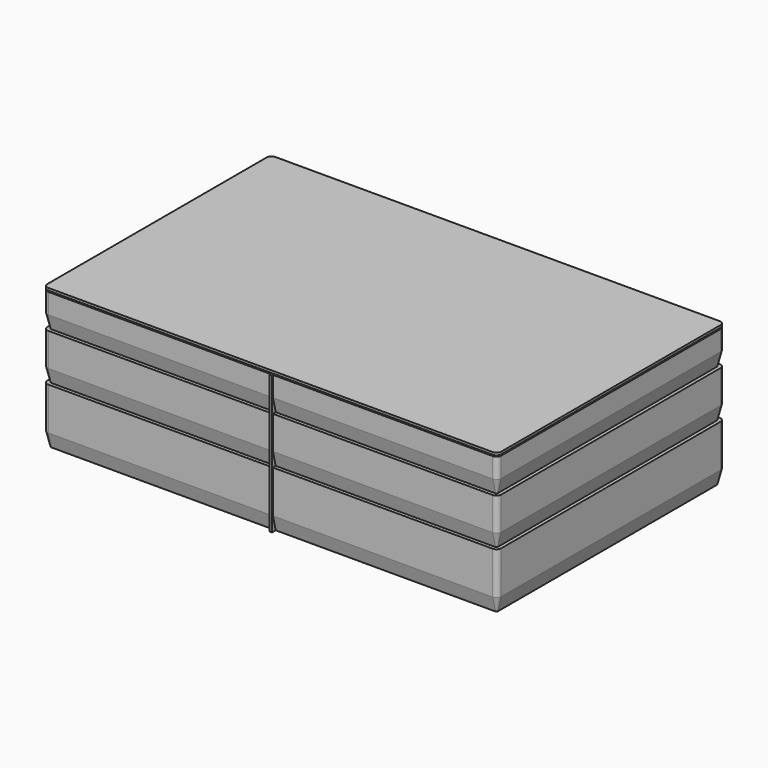
from build123d import *

# Parameters (mm, degrees)
F1_DEPTH = 6.35
F2_START = -9.525
F2_DEPTH = 92.075
F3_SIZE2 = 9.525
F3_SIZE  = 38.1
F4_START = -101.6
F4_DEPTH = 127
F5_SIZE2 = 9.525
F5_SIZE  = 38.1
F6_START = -228.6
F6_DEPTH = 152.4
F7_SIZE2 = 9.525
F7_SIZE  = 38.1
F9_START = -9.525
F8_W     = 6.35
F8_H     = 3.175
F8_H_2   = 19.05
F9_DEPTH = 371.475


# Not quite as in the source:
# - a feature names something its author has since deleted; it is built from what else it names


with BuildPart() as f1:
    # F0 (on Top) → F1 (new body)
    with BuildSketch(Plane.XY):
        with BuildLine():
            Line((39.9490956545, 736.9148339033), (-1153.8509043455, 736.9148339033))
            ThreePointArc((-1153.8509043455, 736.9148339033), (-1162.8311604666, 733.1950900244), (-1166.5509043455, 724.2148339033))
            Line((-1166.5509043455, 724.2148339033), (-1166.5509043455, 40.0023339033))
            Line((-1166.5509043455, 40.0023339033), (-1166.5509043455, 38.4148339033))
            Line((-1166.5509043455, 38.4148339033), (-1147.5009043455, 38.4148339033))
            Line((-1147.5009043455, 38.4148339033), (-1103.0509043455, 38.4148339033))
            Line((-1103.0509043455, 38.4148339033), (-1103.0509043455, -6.0351660967))
            Line((-1103.0509043455, -6.0351660967), (-1103.0509043455, -25.0851660967))
            Line((-1103.0509043455, -25.0851660967), (-1101.4634043455, -25.0851660967))
            Line((-1101.4634043455, -25.0851660967), (-560.1259043455, -25.0851660967))
            Line((-560.1259043455, -25.0851660967), (-553.7759043455, -25.0851660967))
            Line((-553.7759043455, -25.0851660967), (39.9490956545, -25.0851660967))
            ThreePointArc((39.9490956545, -25.0851660967), (48.9293517756, -21.3654222178), (52.6490956545, -12.3851660967))
            Line((52.6490956545, -12.3851660967), (52.6490956545, 724.2148339033))
            ThreePointArc((52.6490956545, 724.2148339033), (48.9293517756, 733.1950900244), (39.9490956545, 736.9148339033))
        make_face()
        with BuildLine():
            Line((-1147.5009043455, 38.4148339033), (-1166.5509043455, 38.4148339033))
            Line((-1166.5509043455, 38.4148339033), (-1166.5509043455, -12.3851660967))
            ThreePointArc((-1166.5509043455, -12.3851660967), (-1162.8311604666, -21.3654222178), (-1153.8509043455, -25.0851660967))
            Line((-1153.8509043455, -25.0851660967), (-1103.0509043455, -25.0851660967))
            Line((-1103.0509043455, -25.0851660967), (-1103.0509043455, -6.0351660967))
            Line((-1103.0509043455, -6.0351660967), (-1103.0509043455, 38.4148339033))
            Line((-1103.0509043455, 38.4148339033), (-1147.5009043455, 38.4148339033))
        make_face()
    extrude(amount=-F1_DEPTH)


with BuildPart() as f2:
    # F0 (on Top) → F2 (new body)
    with BuildSketch(Plane.XY.offset(F2_START)):
        with BuildLine():
            Line((39.9490956545, 736.9148339033), (-1153.8509043455, 736.9148339033))
            ThreePointArc((-1153.8509043455, 736.9148339033), (-1162.8311604666, 733.1950900244), (-1166.5509043455, 724.2148339033))
            Line((-1166.5509043455, 724.2148339033), (-1166.5509043455, 40.0023339033))
            Line((-1166.5509043455, 40.0023339033), (-1166.5509043455, 38.4148339033))
            Line((-1166.5509043455, 38.4148339033), (-1147.5009043455, 38.4148339033))
            Line((-1147.5009043455, 38.4148339033), (-1103.0509043455, 38.4148339033))
            Line((-1103.0509043455, 38.4148339033), (-1103.0509043455, -6.0351660967))
            Line((-1103.0509043455, -6.0351660967), (-1103.0509043455, -25.0851660967))
            Line((-1103.0509043455, -25.0851660967), (-1101.4634043455, -25.0851660967))
            Line((-1101.4634043455, -25.0851660967), (-560.1259043455, -25.0851660967))
            Line((-560.1259043455, -25.0851660967), (-553.7759043455, -25.0851660967))
            Line((-553.7759043455, -25.0851660967), (39.9490956545, -25.0851660967))
            ThreePointArc((39.9490956545, -25.0851660967), (48.9293517756, -21.3654222178), (52.6490956545, -12.3851660967))
            Line((52.6490956545, -12.3851660967), (52.6490956545, 724.2148339033))
            ThreePointArc((52.6490956545, 724.2148339033), (48.9293517756, 733.1950900244), (39.9490956545, 736.9148339033))
        make_face()
        with BuildLine():
            Line((-1147.5009043455, 38.4148339033), (-1166.5509043455, 38.4148339033))
            Line((-1166.5509043455, 38.4148339033), (-1166.5509043455, -12.3851660967))
            ThreePointArc((-1166.5509043455, -12.3851660967), (-1162.8311604666, -21.3654222178), (-1153.8509043455, -25.0851660967))
            Line((-1153.8509043455, -25.0851660967), (-1103.0509043455, -25.0851660967))
            Line((-1103.0509043455, -25.0851660967), (-1103.0509043455, -6.0351660967))
            Line((-1103.0509043455, -6.0351660967), (-1103.0509043455, 38.4148339033))
            Line((-1103.0509043455, 38.4148339033), (-1147.5009043455, 38.4148339033))
        make_face()
    extrude(amount=-F2_DEPTH)

    # F3
    f3_edges = [f2.edges().sort_by_distance(p)[0] for p in [
        (-556.950904, 736.914834, -101.6),
        (-1162.83116, 733.19509, -101.6),
        (-1166.550904, 355.914834, -101.6),
        (-1162.83116, -21.365422, -101.6),
        (-556.950904, -25.085166, -101.6),
        (48.929352, -21.365422, -101.6),
        (52.649096, 355.914834, -101.6),
        (48.929352, 733.19509, -101.6),
    ]]
    chamfer(f3_edges, length=F3_SIZE, length2=F3_SIZE2)

    # F0 (on Top) → F4 (join)
    with BuildSketch(Plane.XY.offset(F4_START)):
        with BuildLine():
            Line((39.9490956545, 736.9148339033), (-1153.8509043455, 736.9148339033))
            ThreePointArc((-1153.8509043455, 736.9148339033), (-1162.8311604666, 733.1950900244), (-1166.5509043455, 724.2148339033))
            Line((-1166.5509043455, 724.2148339033), (-1166.5509043455, 40.0023339033))
            Line((-1166.5509043455, 40.0023339033), (-1166.5509043455, 38.4148339033))
            Line((-1166.5509043455, 38.4148339033), (-1147.5009043455, 38.4148339033))
            Line((-1147.5009043455, 38.4148339033), (-1103.0509043455, 38.4148339033))
            Line((-1103.0509043455, 38.4148339033), (-1103.0509043455, -6.0351660967))
            Line((-1103.0509043455, -6.0351660967), (-1103.0509043455, -25.0851660967))
            Line((-1103.0509043455, -25.0851660967), (-1101.4634043455, -25.0851660967))
            Line((-1101.4634043455, -25.0851660967), (-560.1259043455, -25.0851660967))
            Line((-560.1259043455, -25.0851660967), (-553.7759043455, -25.0851660967))
            Line((-553.7759043455, -25.0851660967), (39.9490956545, -25.0851660967))
            ThreePointArc((39.9490956545, -25.0851660967), (48.9293517756, -21.3654222178), (52.6490956545, -12.3851660967))
            Line((52.6490956545, -12.3851660967), (52.6490956545, 724.2148339033))
            ThreePointArc((52.6490956545, 724.2148339033), (48.9293517756, 733.1950900244), (39.9490956545, 736.9148339033))
        make_face()
        with BuildLine():
            Line((-1147.5009043455, 38.4148339033), (-1166.5509043455, 38.4148339033))
            Line((-1166.5509043455, 38.4148339033), (-1166.5509043455, -12.3851660967))
            ThreePointArc((-1166.5509043455, -12.3851660967), (-1162.8311604666, -21.3654222178), (-1153.8509043455, -25.0851660967))
            Line((-1153.8509043455, -25.0851660967), (-1103.0509043455, -25.0851660967))
            Line((-1103.0509043455, -25.0851660967), (-1103.0509043455, -6.0351660967))
            Line((-1103.0509043455, -6.0351660967), (-1103.0509043455, 38.4148339033))
            Line((-1103.0509043455, 38.4148339033), (-1147.5009043455, 38.4148339033))
        make_face()
    extrude(amount=-F4_DEPTH)

    # F5
    f5_edges = [f2.edges().sort_by_distance(p)[0] for p in [
        (-556.950904, 736.914834, -228.6),
        (-1162.83116, 733.19509, -228.6),
        (-1166.550904, 355.914834, -228.6),
        (-1162.83116, -21.365422, -228.6),
        (-556.950904, -25.085166, -228.6),
        (48.929352, -21.365422, -228.6),
        (52.649096, 355.914834, -228.6),
        (48.929352, 733.19509, -228.6),
    ]]
    chamfer(f5_edges, length=F5_SIZE, length2=F5_SIZE2)

    # F0 (on Top) → F6 (join)
    with BuildSketch(Plane.XY.offset(F6_START)):
        with BuildLine():
            Line((39.9490956545, 736.9148339033), (-1153.8509043455, 736.9148339033))
            ThreePointArc((-1153.8509043455, 736.9148339033), (-1162.8311604666, 733.1950900244), (-1166.5509043455, 724.2148339033))
            Line((-1166.5509043455, 724.2148339033), (-1166.5509043455, 40.0023339033))
            Line((-1166.5509043455, 40.0023339033), (-1166.5509043455, 38.4148339033))
            Line((-1166.5509043455, 38.4148339033), (-1147.5009043455, 38.4148339033))
            Line((-1147.5009043455, 38.4148339033), (-1103.0509043455, 38.4148339033))
            Line((-1103.0509043455, 38.4148339033), (-1103.0509043455, -6.0351660967))
            Line((-1103.0509043455, -6.0351660967), (-1103.0509043455, -25.0851660967))
            Line((-1103.0509043455, -25.0851660967), (-1101.4634043455, -25.0851660967))
            Line((-1101.4634043455, -25.0851660967), (-560.1259043455, -25.0851660967))
            Line((-560.1259043455, -25.0851660967), (-553.7759043455, -25.0851660967))
            Line((-553.7759043455, -25.0851660967), (39.9490956545, -25.0851660967))
            ThreePointArc((39.9490956545, -25.0851660967), (48.9293517756, -21.3654222178), (52.6490956545, -12.3851660967))
            Line((52.6490956545, -12.3851660967), (52.6490956545, 724.2148339033))
            ThreePointArc((52.6490956545, 724.2148339033), (48.9293517756, 733.1950900244), (39.9490956545, 736.9148339033))
        make_face()
        with BuildLine():
            Line((-1147.5009043455, 38.4148339033), (-1166.5509043455, 38.4148339033))
            Line((-1166.5509043455, 38.4148339033), (-1166.5509043455, -12.3851660967))
            ThreePointArc((-1166.5509043455, -12.3851660967), (-1162.8311604666, -21.3654222178), (-1153.8509043455, -25.0851660967))
            Line((-1153.8509043455, -25.0851660967), (-1103.0509043455, -25.0851660967))
            Line((-1103.0509043455, -25.0851660967), (-1103.0509043455, -6.0351660967))
            Line((-1103.0509043455, -6.0351660967), (-1103.0509043455, 38.4148339033))
            Line((-1103.0509043455, 38.4148339033), (-1147.5009043455, 38.4148339033))
        make_face()
    extrude(amount=-F6_DEPTH)

    # F7
    f7_edges = [f2.edges().sort_by_distance(p)[0] for p in [
        (-556.950904, 736.914834, -381),
        (-1162.83116, 733.19509, -381),
        (-1166.550904, 355.914834, -381),
        (-1162.83116, -21.365422, -381),
        (-556.950904, -25.085166, -381),
        (48.929352, -21.365422, -381),
        (52.649096, 355.914834, -381),
        (48.929352, 733.19509, -381),
    ]]
    chamfer(f7_edges, length=F7_SIZE, length2=F7_SIZE2)


with BuildPart() as f9:
    # F8 (on face) → F9 (new body)
    with BuildSketch(Plane.XY.offset(F9_START)):
        with Locations((-553.7759043455, -26.6726660967)):
            Rectangle(F8_W, F8_H)
        with Locations((-553.7759043455, -15.5601660967)):
            Rectangle(F8_W, F8_H_2)
    extrude(amount=-F9_DEPTH)


solid = Compound([f1.part, f2.part, f9.part])
